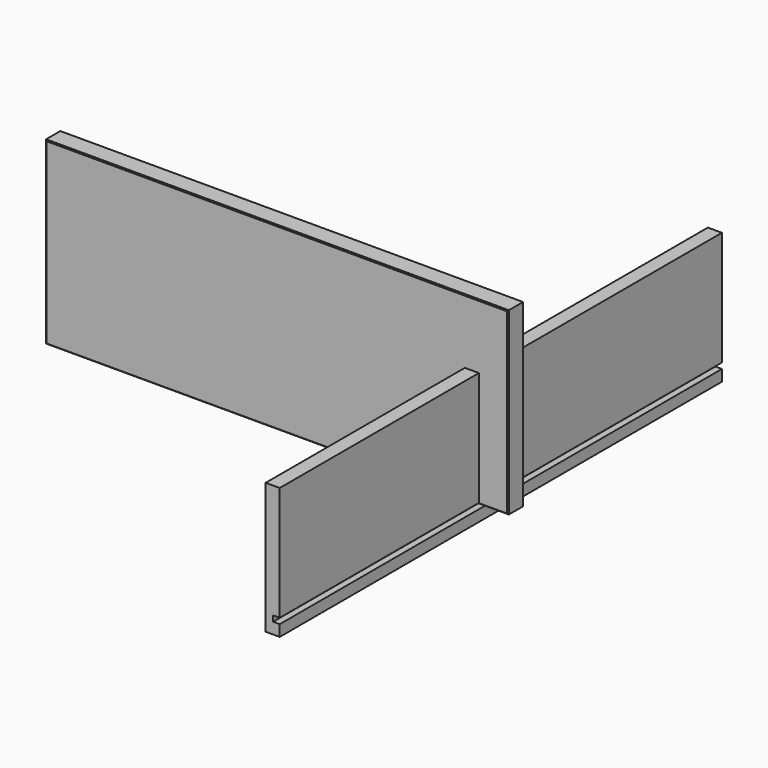
from build123d import *

# Parameters (mm, degrees)
F0_W     = 494
F0_H     = 192
F1_DEPTH = 20
F2_SIZE  = 1
F3_W     = 590
F3_H     = 140
F4_DEPTH = 15
F5_W     = 15
F5_H     = 6
F6_DEPTH = 800


with BuildPart() as f1:
    # F0 (on Front) → F1 (new body)
    with BuildSketch(Plane.XZ):
        with Locations((-200.8205638528, 72.6834676266)):
            Rectangle(F0_W, F0_H)
    extrude(amount=F1_DEPTH)

    # F2
    f2_edges = [f1.edges().sort_by_distance(p)[0] for p in [
        (-200.820564, -20, -23.316532),
        (46.179436, -20, 72.683468),
        (-200.820564, -20, 168.683468),
        (-447.820564, -20, 72.683468),
    ]]
    chamfer(f2_edges, length=F2_SIZE)


with BuildPart() as f4:
    # F3 (on Right) → F4 (new body)
    with BuildSketch(Plane.YZ):
        with Locations((9.2540290207, 29.9439153292)):
            Rectangle(F3_W, F3_H)
    extrude(amount=F4_DEPTH)

    # F5 (on face) → F6 (cut)
    with BuildSketch(Plane.XZ.offset(285.7459709793)):
        with Locations((15.5, -25.0560846708)):
            Rectangle(F5_W, F5_H)
    extrude(amount=-F6_DEPTH, mode=Mode.SUBTRACT)


solid = Compound([f1.part, f4.part])
